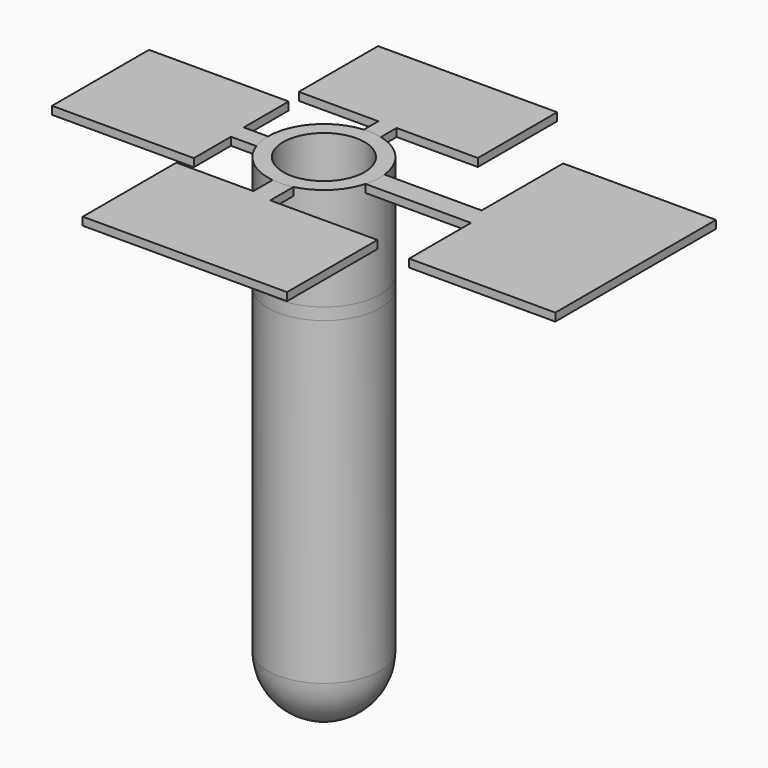
from build123d import *

# Parameters (mm, degrees)
F0_R      = 7
F1_DEPTH  = 7
F2_R      = 6.99999
F4_DEPTH  = 40
F5_R      = 7
F5_R_2    = 5.75
F6_DEPTH  = 1.5
F7_R      = 7
F7_R_2    = 5.1
F8_DEPTH  = 12.9
F10_DEPTH = 1


# Not quite as in the source:
# - a fillet or chamfer is up to 0.001 mm smaller than in the source, because OpenCascade refuses the exact size


with BuildPart() as f1:
    # F0 (on Top) → F1 (new body)
    with BuildSketch(Plane.XY):
        Circle(F0_R)
        with BuildLine():
            ThreePointArc((-5.75, 0), (0, 5.75), (5.75, 0))
            ThreePointArc((5.75, 0), (0, -5.75), (-5.75, 0))
        make_face(mode=Mode.SUBTRACT)
        with BuildLine():
            Line((-5.75, 0), (5.75, 0))
            ThreePointArc((5.75, 0), (0, 5.75), (-5.75, 0))
        make_face()
        with BuildLine():
            ThreePointArc((-5.75, 0), (0, -5.75), (5.75, 0))
            Line((5.75, 0), (-5.75, 0))
        make_face()
    extrude(amount=-F1_DEPTH)

    # F2 (radius 7 in the source; OpenCascade refuses exactly that, so slightly less here)
    f2_edges = [f1.edges().sort_by_distance(p)[0] for p in [
        (-7, 0, -7),
    ]]
    fillet(f2_edges, radius=F2_R)

    # F0 (on Top) → F3 (revolve, cut)
    with BuildSketch(Plane.XY):
        with BuildLine():
            ThreePointArc((-5.75, 0), (0, -5.75), (5.75, 0))
            Line((5.75, 0), (-5.75, 0))
        make_face()
    revolve(axis=Axis((0, 0, 0), (1, 0, 0)), mode=Mode.SUBTRACT)

    # F4 (add): a face of the model
    f4_faces = [f1.faces().sort_by_distance(p)[0] for p in [
        (-6.8020101013, 0, 0),
    ]]
    extrude(f4_faces, amount=F4_DEPTH)

    # F5 (on face) → F6 (join)
    with BuildSketch(Plane.XY.offset(40)):
        Circle(F5_R)
        Circle(F5_R_2, mode=Mode.SUBTRACT)
        Circle(F5_R_2)
    extrude(amount=F6_DEPTH)

    # F7 (on face) → F8 (join)
    with BuildSketch(Plane.XY.offset(41.5)):
        Circle(F7_R)
        Circle(F7_R_2, mode=Mode.SUBTRACT)
    extrude(amount=F8_DEPTH)

    # F9 (on face) → F10 (join)
    with BuildSketch(Plane.XY.offset(54.4)):
        with BuildLine():
            ThreePointArc((-6.6038061512, -2.3215822875), (-6.9002406863, -1.1775731276), (-7, 0))
            Line((-7, 0), (-10.0409816951, 0))
            Line((-10.0409816951, 0), (-10.0409816951, 7.0408415049))
            Line((-10.0409816951, 7.0408415049), (-27.5440905243, 7.0408415049))
            Line((-27.5440905243, 7.0408415049), (-27.5440905243, -6.5598203801))
            Line((-27.5440905243, -6.5598203801), (-27.5440905243, -8.1330426037))
            Line((-27.5440905243, -8.1330426037), (-9.7872372717, -8.1330426037))
            Line((-9.7872372717, -8.1330426037), (-9.7872372717, -2.3215822875))
            Line((-9.7872372717, -2.3215822875), (-6.6038061512, -2.3215822875))
        make_face()
        with BuildLine():
            Line((-0.5746171277, 9.2485286327), (-0.5746171277, 6.9763755028))
            ThreePointArc((-0.5746171277, 6.9763755028), (0.5741414209, 6.9764146686), (1.7074374482, 6.7885681377))
            Line((1.7074374482, 6.7885681377), (1.7074374482, 9.2485286327))
            Line((1.7074374482, 9.2485286327), (11.8826339021, 9.2485286327))
            Line((11.8826339021, 9.2485286327), (11.8826339021, 21.6566864401))
            Line((11.8826339021, 21.6566864401), (-10.5484733358, 21.6566864401))
            Line((-10.5484733358, 21.6566864401), (-10.5484733358, 9.2485286327))
            Line((-10.5484733358, 9.2485286327), (-7.0214094594, 9.2485286327))
            Line((-7.0214094594, 9.2485286327), (-0.5746171277, 9.2485286327))
        make_face()
        with BuildLine():
            Line((14.655204518, 0.8017900982), (6.9539292949, 0.8017900982))
            ThreePointArc((6.9539292949, 0.8017900982), (6.9884728326, 0.4015563072), (7, 0))
            ThreePointArc((7, 0), (6.9335784443, -0.9620238859), (6.735574298, -1.9057908794))
            Line((6.735574298, -1.9057908794), (19.9458785355, -1.9057908794))
            Line((19.9458785355, -1.9057908794), (19.9458785355, -11.5896631032))
            Line((19.9458785355, -11.5896631032), (38.256034255, -11.5896631032))
            Line((38.256034255, -11.5896631032), (38.256034255, 13.5597093031))
            Line((38.256034255, 13.5597093031), (19.1134941834, 13.5597093031))
            Line((19.1134941834, 13.5597093031), (19.1134941834, 0.8017900982))
            Line((19.1134941834, 0.8017900982), (14.655204518, 0.8017900982))
        make_face()
        with BuildLine():
            ThreePointArc((1.6340564471, -6.8066041113), (0.3847522235, -6.989418125), (-0.8770696547, -6.9448361263))
            Line((-0.8770696547, -6.9448361263), (-0.8770696547, -9.9506975346))
            Line((-0.8770696547, -9.9506975346), (-10.5280578136, -9.9506975346))
            Line((-10.5280578136, -9.9506975346), (-10.5280578136, -24.5994888246))
            Line((-10.5280578136, -24.5994888246), (15.0621160865, -24.5994888246))
            Line((15.0621160865, -24.5994888246), (15.0621160865, -10.4480329901))
            Line((15.0621160865, -10.4480329901), (1.6340564471, -10.4480329901))
            Line((1.6340564471, -10.4480329901), (1.6340564471, -6.8066041113))
        make_face()
    extrude(amount=-F10_DEPTH)


solid = f1.part
